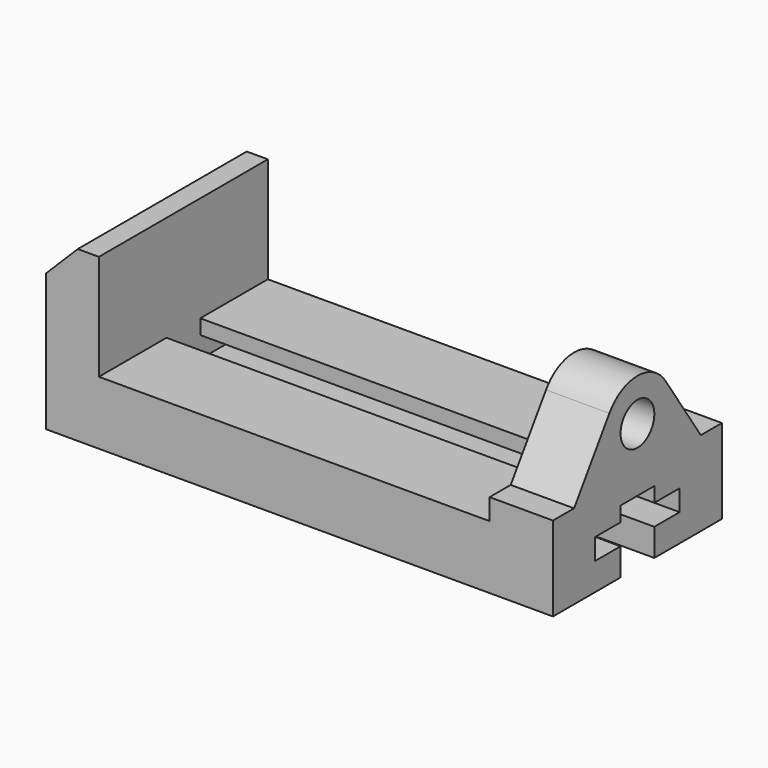
from build123d import *

# Parameters (mm, degrees)
F0_R     = 12.7
F1_DEPTH = 38.1
F3_DEPTH = 127
F5_DEPTH = 273.05


# Not quite as in the source:
# - a feature names something its author has since deleted; it is built from what else it names


with BuildPart() as f1:
    # F0 (on Right) → F1 (new body)
    with BuildSketch(Plane.YZ):
        with BuildLine():
            Line((0, 50.8), (0, 0))
            Line((0, 0), (127, 0))
            Line((127, 0), (127, 50.8))
            Line((127, 50.8), (111.125, 50.8))
            Line((111.125, 50.8), (84.5934256055, 90.3501730104))
            ThreePointArc((84.5934256055, 90.3501730104), (63.5, 101.6), (42.4065743945, 90.3501730104))
            Line((42.4065743945, 90.3501730104), (15.875, 50.8))
            Line((15.875, 50.8), (0, 50.8))
        make_face()
        with Locations((63.5, 76.2)):
            Circle(F0_R, mode=Mode.SUBTRACT)
    extrude(amount=F1_DEPTH)

    # F2 (on face) → F3 (join)
    with BuildSketch(Plane.XZ):
        Polygon((0, 0), (0, 38.1), (-234.95, 38.1), (-234.95, 101.6), (-247.65, 101.6), (-266.7, 82.55), (-266.7, 0), align=None)
    extrude(amount=-F3_DEPTH)

    # F4 (on face) → F5 (cut)
    with BuildSketch(Plane.YZ.offset(38.1)):
        Polygon((50.8, 0), (63.5, 0), (76.2, 0), (76.2, 16.51), (95.25, 16.51), (95.25, 29.21), (76.2, 29.21), (76.2, 38.1), (50.8, 38.1), (50.8, 29.21), (31.75, 29.21), (31.75, 16.51), (50.8, 16.51), align=None)
    extrude(amount=-F5_DEPTH, mode=Mode.SUBTRACT)


solid = f1.part
